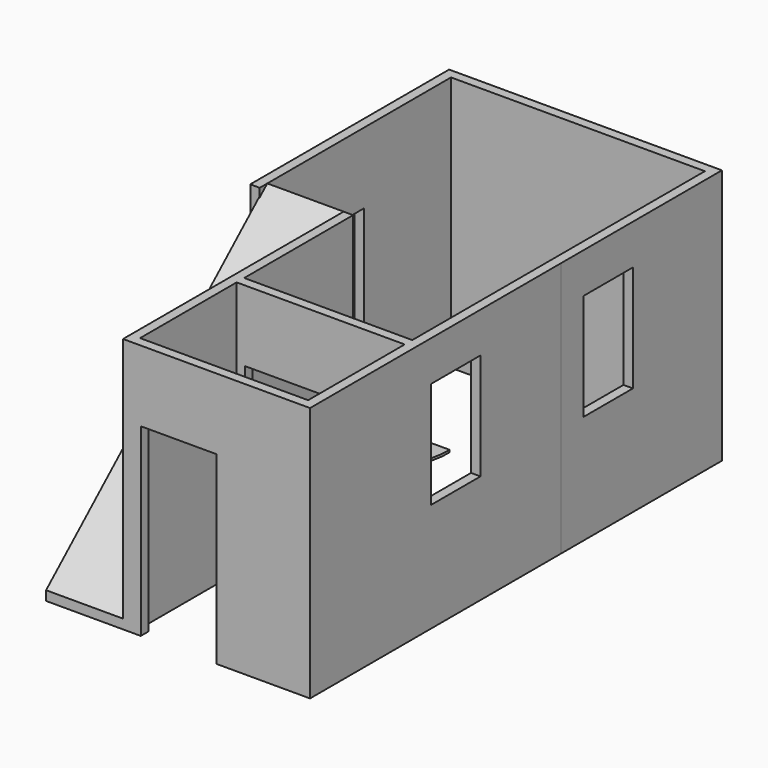
from build123d import *

# Parameters (mm, degrees)
F0_W      = 1803.4
F0_H      = 1295.4
F1_DEPTH  = 2743.2
F2_W      = 812.8
F2_H      = 1981.2
F3_DEPTH  = 3606.8
F4_W      = 914.4
F4_H      = 1981.2
F5_DEPTH  = 101.6
F6_W      = 660.4
F6_H      = 1143
F7_DEPTH  = 101.6
F8_W      = 660.4
F8_H      = 1143
F9_DEPTH  = 101.6
F11_DEPTH = 25.4
F13_DEPTH = 825.5


# Not quite as in the source:
# - ends of sketch curves that miss each other by under 0.0002 mm in the source are joined


with BuildPart() as f1:
    # F0 (on Top) → F1 (new body)
    with BuildSketch(Plane.XY):
        Polygon((901.7, 3740.1499866486), (901.7, 1682.7499866486), (901.7, 1581.15), (901.7, -184.15), (-901.7, -184.15), (-901.7, 1276.3499866486), (-1003.2999866486, 1276.3499866486), (-1003.2999866486, -1682.7499866486), (1003.2999866486, -1682.7499866486), (1003.2999866486, 1682.7499866486), (1003.3, 3841.7499866486), (-1924.05, 3841.7499866486), (-1924.05, 1174.7499866486), (-1822.45, 1174.7499866486), (-1822.45, 3740.1499866486), align=None)
        with Locations((0, -933.45)):
            Rectangle(F0_W, F0_H, mode=Mode.SUBTRACT)
    extrude(amount=F1_DEPTH)

    # F2 (on face) → F3 (cut)
    with BuildSketch(Plane.XZ.offset(1682.7499866486)):
        with Locations((-406.4, 990.6)):
            Rectangle(F2_W, F2_H)
    extrude(amount=-F3_DEPTH, mode=Mode.SUBTRACT)

    # F4 (on face) → F5 (cut)
    with BuildSketch(Plane(origin=(-1924.05, 0, 0), x_dir=(0, -1, 0), z_dir=(-1, 0, 0))):
        with Locations((-2114.073614502, 990.6)):
            Rectangle(F4_W, F4_H)
    extrude(amount=-F5_DEPTH, mode=Mode.SUBTRACT)

    # F6 (on face) → F7 (cut)
    with BuildSketch(Plane.YZ.offset(1003.2999866486)):
        with Locations((273.0499866486, 1739.9)):
            Rectangle(F6_W, F6_H)
    extrude(amount=-F7_DEPTH, mode=Mode.SUBTRACT)

    # F8 (on face) → F9 (cut)
    with BuildSketch(Plane.YZ.offset(1003.3)):
        with Locations((2317.7499866486, 1739.9)):
            Rectangle(F8_W, F8_H)
    extrude(amount=-F9_DEPTH, mode=Mode.SUBTRACT)

    # F10 (on face) → F11 (join)
    with BuildSketch(Plane(origin=(0, 0, 0), x_dir=(1, 0, 0), z_dir=(0, 0, -1))):
        with BuildLine():
            Line((-1822.45, -1650.6354808807), (-1822.45, -2571.273614502))
            Line((-1822.45, -2571.273614502), (-901.8118663788, -2571.273614502))
            ThreePointArc((-901.8118663788, -2571.273614502), (-1171.4605326975, -1920.2841471995), (-1822.45, -1650.6354808807))
        make_face()
    extrude(amount=F11_DEPTH)

    # F12 (on face) → F13 (join)
    with BuildSketch(Plane(origin=(-1003.2999866486, 0, 0), x_dir=(0, -1, 0), z_dir=(-1, 0, 0))):
        Polygon((1682.7499866486, 101.6), (-1276.3499866486, 2743.2), (-1276.3499866486, 2641.6), (1682.7499866486, 0), align=None)
    extrude(amount=F13_DEPTH)


solid = f1.part
